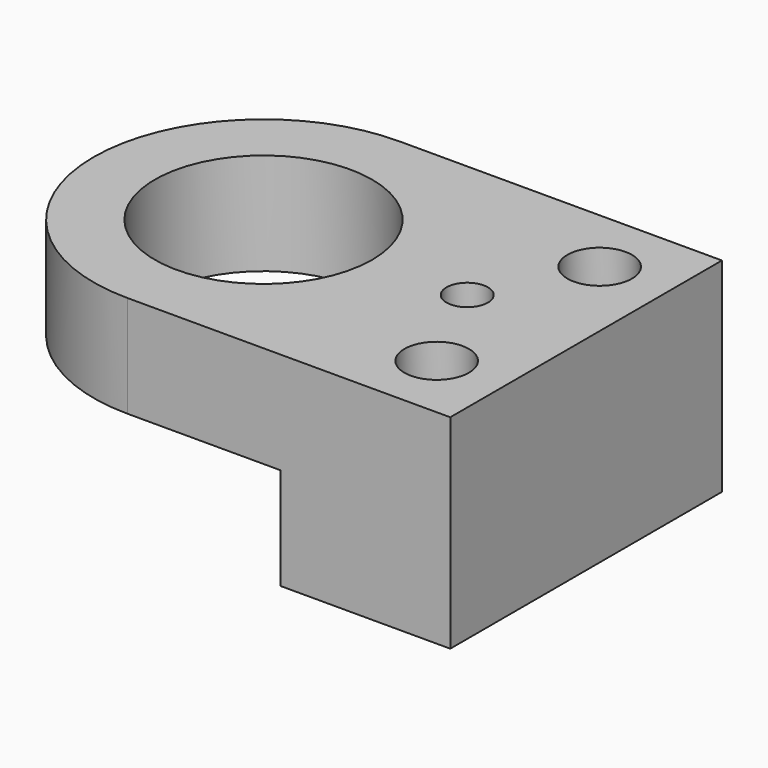
from build123d import *

# Parameters (mm, degrees)
F0_W            = 72.5
F0_H            = 50
F1_DEPTH        = 30
F2_R            = 16
F3_DEPTH        = 30.001
F5_D            = 6.1
F5_DEPTH        = 8
F5_TIP          = 1.832624888
F6_R            = 32.5
F7_DEPTH        = 15
F8_R            = 24.99999
F10_D           = 5.5
F10_CBORE_D     = 9.5
F10_CBORE_DEPTH = 5
F11_W           = 1.7334403427
F11_H           = 15
F12_DEPTH       = 50.001


# Not quite as in the source:
# - a fillet or chamfer is up to 0.001 mm smaller than in the source, because OpenCascade refuses the exact size


with BuildPart() as f1:
    # F0 (on Top) → F1 (new body)
    with BuildSketch(Plane.XY):
        with Locations((-18.75, 0)):
            Rectangle(F0_W, F0_H)
    extrude(amount=F1_DEPTH)

    # F2 (on face) → F3 (cut, through all)
    with BuildSketch(Plane.XY.offset(30)):
        with Locations((-30, 0)):
            Circle(F2_R)
    extrude(amount=-F3_DEPTH, mode=Mode.SUBTRACT)

    # F5
    with Locations(Plane.XY.offset(30)):
        with Locations((0, 0)):
            Hole(F5_D / 2, depth=F5_DEPTH)
            with Locations((0, 0, -(F5_DEPTH + F5_TIP / 2))):  # 118° drill point
                Cone(0, F5_D / 2, F5_TIP, mode=Mode.SUBTRACT)

    # F6 (on face) → F7 (cut)
    with BuildSketch(Plane(origin=(0, 0, 0), x_dir=(1, 0, 0), z_dir=(0, 0, -1))):
        with Locations((-30, 0)):
            Circle(F6_R)
    extrude(amount=-F7_DEPTH, mode=Mode.SUBTRACT)

    # F8 (radius 25 in the source; OpenCascade refuses exactly that, so slightly less here)
    f8_edges = [f1.edges().sort_by_distance(p)[0] for p in [
        (-55, -25, 15),
        (-55, 25, 15),
    ]]
    fillet(f8_edges, radius=F8_R)

    # F10 (through all)
    with Locations(Plane.XY.offset(30)):
        with Locations((7.5, 15), (7.5, -15)):
            CounterBoreHole(F10_D / 2, F10_CBORE_D / 2, F10_CBORE_DEPTH)

    # F11 (on face) → F12 (cut, through all)
    with BuildSketch(Plane(origin=(0, 25, 0), x_dir=(-1, 0, 0), z_dir=(0, 1, 0))):
        with Locations((8.3667201714, 7.5)):
            Rectangle(F11_W, F11_H)
    extrude(amount=-F12_DEPTH, mode=Mode.SUBTRACT)


solid = f1.part
